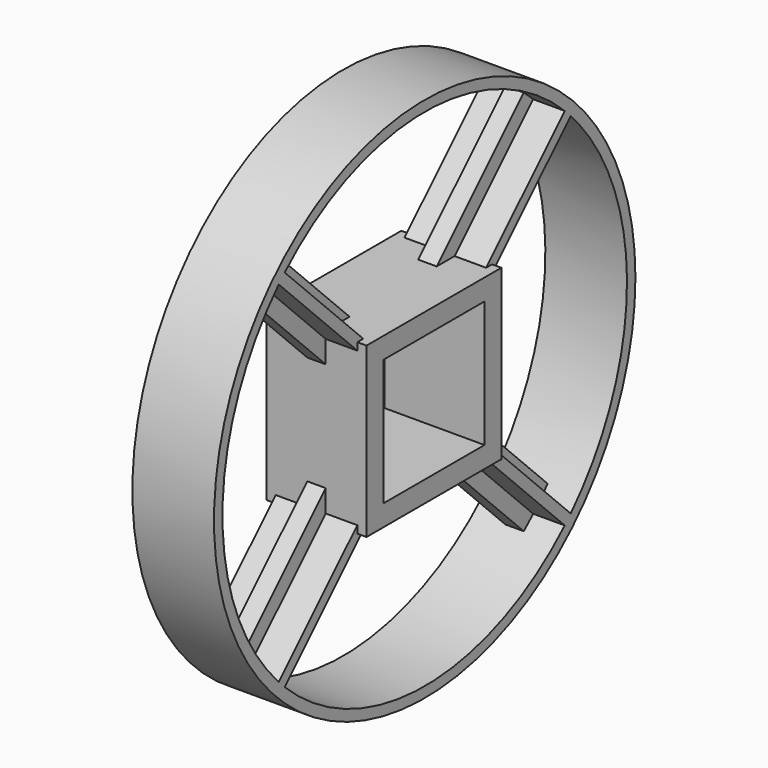
from build123d import *

# Parameters (mm, degrees)
F0_W            = 152.4
F0_H            = 152.4
F1_DEPTH        = 60.325
F2_DEPTH        = 49.2125
F2_COPIES_COUNT = 4
F3_DEPTH        = 11.1125
F3_COPIES_COUNT = 4
F0_R            = 317.5
F4_DEPTH        = 49.2125


# Not quite as in the source:
# - a pattern or mirror of a feature is missing from the dataset's text; its kind, count and spacing are read off the source's solid


with BuildPart() as f1:
    # F0 (on Right) → F1 (new body, symmetric)
    with BuildSketch(Plane.YZ):
        Polygon((101.6, -101.6), (101.6, 65.6789755157), (101.6, 92.6197438789), (101.6, 101.6), (92.6197438789, 101.6), (65.6789755157, 101.6), (-101.6, 101.6), (-101.6, -101.6), align=None)
        Rectangle(F0_W, F0_H, mode=Mode.SUBTRACT)
    extrude(amount=F1_DEPTH, both=True)

    # F0 (on Right) → F2 (join, symmetric)
    with BuildSketch(Plane.YZ):
        with BuildLine():
            Line((101.6, 92.6197438789), (219.9694977227, 210.9892416016))
            ThreePointArc((219.9694977227, 210.9892416016), (215.5261469057, 215.5261469057), (210.9892416016, 219.9694977227))
            Line((210.9892416016, 219.9694977227), (92.6197438789, 101.6))
            Line((92.6197438789, 101.6), (101.6, 101.6))
            Line((101.6, 101.6), (101.6, 92.6197438789))
        make_face()
    f2 = extrude(amount=F2_DEPTH, both=True)

    # F2_copies: F2 ×4 about axis
    f2_copies_axis = Axis((0, 0, 0), (1, 0, 0))
    for i in range(1, F2_COPIES_COUNT):
        add(f2.rotate(f2_copies_axis, i * 360 / F2_COPIES_COUNT))

    # F0 (on Right) → F3 (join, symmetric)
    with BuildSketch(Plane.YZ):
        with BuildLine():
            ThreePointArc((210.9892416016, 219.9694977227), (204.0025151944, 226.4641556502), (196.815976229, 232.7370007133))
            Line((196.815976229, 232.7370007133), (65.6789755157, 101.6))
            Line((65.6789755157, 101.6), (92.6197438789, 101.6))
            Line((92.6197438789, 101.6), (210.9892416016, 219.9694977227))
        make_face()
        with BuildLine():
            Line((101.6, 65.6789755157), (232.7370007133, 196.815976229))
            ThreePointArc((232.7370007133, 196.815976229), (226.4641556502, 204.0025151944), (219.9694977227, 210.9892416016))
            Line((219.9694977227, 210.9892416016), (101.6, 92.6197438789))
            Line((101.6, 92.6197438789), (101.6, 65.6789755157))
        make_face()
    f3 = extrude(amount=F3_DEPTH, both=True)

    # F3_copies: F3 ×4 about axis
    f3_copies_axis = Axis((0, 0, 0), (1, 0, 0))
    for i in range(1, F3_COPIES_COUNT):
        add(f3.rotate(f3_copies_axis, i * 360 / F3_COPIES_COUNT))

    # F0 (on Right) → F4 (join, symmetric)
    with BuildSketch(Plane.YZ):
        Circle(F0_R)
        with BuildLine():
            ThreePointArc((232.7370007133, 196.815976229), (286.2178172454, 104.7969517271), (304.8, 0))
            ThreePointArc((304.8, 0), (-276.4891946845, -128.2839242567), (196.815976229, 232.7370007133))
            ThreePointArc((196.815976229, 232.7370007133), (204.0025151944, 226.4641556502), (210.9892416016, 219.9694977227))
            ThreePointArc((210.9892416016, 219.9694977227), (215.5261469057, 215.5261469057), (219.9694977227, 210.9892416016))
            ThreePointArc((219.9694977227, 210.9892416016), (226.4641556502, 204.0025151944), (232.7370007133, 196.815976229))
        make_face(mode=Mode.SUBTRACT)
    extrude(amount=F4_DEPTH, both=True)


solid = f1.part
